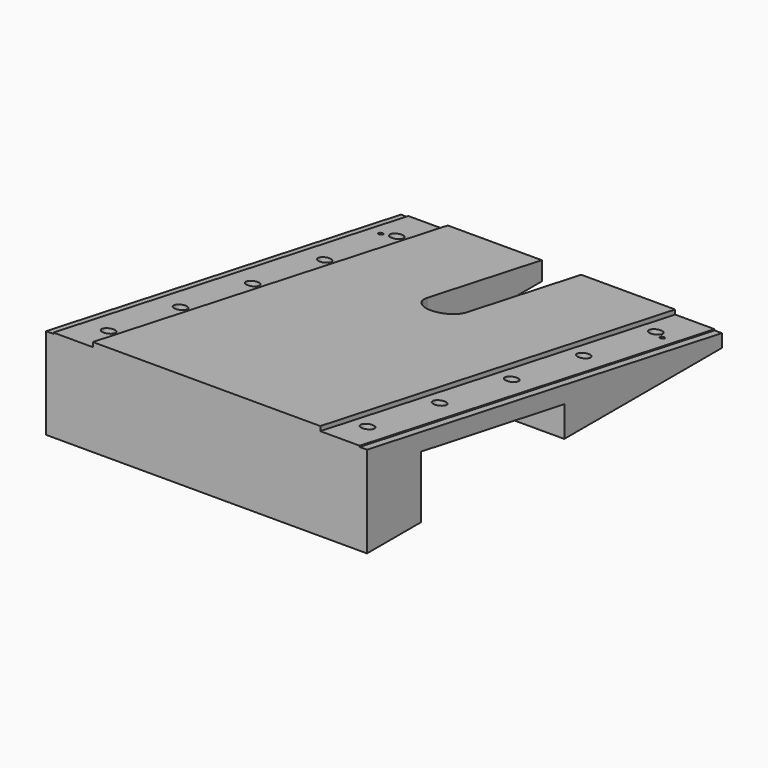
from build123d import *

# Parameters (mm, degrees)
F1_DEPTH  = 285
F3_DEPTH  = 41.5
F5_DEPTH  = 6.5
F7_DEPTH  = 41.5
F8_DEPTH  = 6.5
F13_D     = 11
F15_D     = 13.5
F15_DEPTH = 18
F15_START = 0.4782643
F15_TIP   = 4.0558091784
F17_DEPTH = 85.6227357069
F19_D     = 10
F19_DEPTH = 12
F19_TIP   = 3.0043030951


# Not quite as in the source:
# - a feature names something its author has since deleted; it is built from what else it names


with BuildPart() as f1:
    # F0 (on Right) → F1 (new body)
    with BuildSketch(Plane.YZ):
        Polygon((60, 55.2), (0, 65.8), (0, 0), (60, 0), align=None)
        Polygon((394, 17.0782642931), (0, 86.1), (0, 65.8), (60, 55.2), (219, 27.6782642931), (219, 0.4782642931), (394, 0.4782642931), align=None)
    extrude(amount=-F1_DEPTH)

    # F2 (on face) → F3 (cut)
    with BuildSketch(Plane.YZ):
        Polygon((394, 17.0782642931), (0, 86.1), (0, 82.1), (394, 13.0782642931), align=None)
    extrude(amount=-F3_DEPTH, mode=Mode.SUBTRACT)

    # F4 (on face) → F5 (cut)
    with BuildSketch(Plane.YZ):
        Polygon((394, 13.0782642931), (0, 82.1), (0, 81.1), (394, 12.0782642931), align=None)
    extrude(amount=-F5_DEPTH, mode=Mode.SUBTRACT)

    # F6 (on face) → F7 (cut)
    with BuildSketch(Plane(origin=(-285, 0, 0), x_dir=(0, -1, 0), z_dir=(-1, 0, 0))):
        Polygon((0, 86.1), (-394, 17.0782642931), (-394, 13.0782642931), (0, 82.1), align=None)
    extrude(amount=-F7_DEPTH, mode=Mode.SUBTRACT)

    # F6 (on face) → F8 (cut)
    with BuildSketch(Plane(origin=(-285, 0, 0), x_dir=(0, -1, 0), z_dir=(-1, 0, 0))):
        Polygon((0, 82.1), (-394, 13.0782642931), (-394, 12.0782642931), (0, 81.1), align=None)
    extrude(amount=-F8_DEPTH, mode=Mode.SUBTRACT)

    # F13 (through all)
    with Locations(Plane.XY.offset(86.1)):
        with Locations((-257.5, 355), (-257.5, 275), (-257.5, 195), (-27.5, 355), (-27.5, 275), (-27.5, 195), (-27.5, 115), (-27.5, 35), (-257.5, 115), (-257.5, 35)):
            Hole(F13_D / 2)

    # F15
    # its depths count from where the whole tool has entered the part; down to there all is cleared
    with Locations(Plane(origin=(0, 0, 0), x_dir=(1, 0, 0), z_dir=(0, 0, -1))):
        with Locations((-17.5, -349, 0), (-17.5, -264, -F15_START), (-17.5, -30, 0), (-267.5, -30, 0), (-267.5, -264, -F15_START), (-267.5, -349, 0)):
            Hole(F15_D / 2, depth=F15_DEPTH)
            with Locations((0, 0, -(F15_DEPTH + F15_TIP / 2))):  # 118° drill point
                Cone(0, F15_D / 2, F15_TIP, mode=Mode.SUBTRACT)

    # F16 (on face) → F17 (cut, through all)
    with BuildSketch(Plane(origin=(0, 0, 0.4782642931), x_dir=(1, 0, 0), z_dir=(0, 0, -1))):
        with BuildLine():
            Line((-160, -394), (-125, -394))
            Line((-125, -394), (-125, -266.5))
            ThreePointArc((-125, -266.5), (-142.5, -249), (-160, -266.5))
            Line((-160, -266.5), (-160, -394))
        make_face()
    extrude(amount=-F17_DEPTH, mode=Mode.SUBTRACT)

    # F19
    with Locations(Plane(origin=(0, 0, 0.4782642931), x_dir=(1, 0, 0), z_dir=(0, 0, -1))):
        with Locations((-142.5, -239)):
            Hole(F19_D / 2, depth=F19_DEPTH)
            with Locations((0, 0, -(F19_DEPTH + F19_TIP / 2))):  # 118° drill point
                Cone(0, F19_D / 2, F19_TIP, mode=Mode.SUBTRACT)


solid = f1.part
